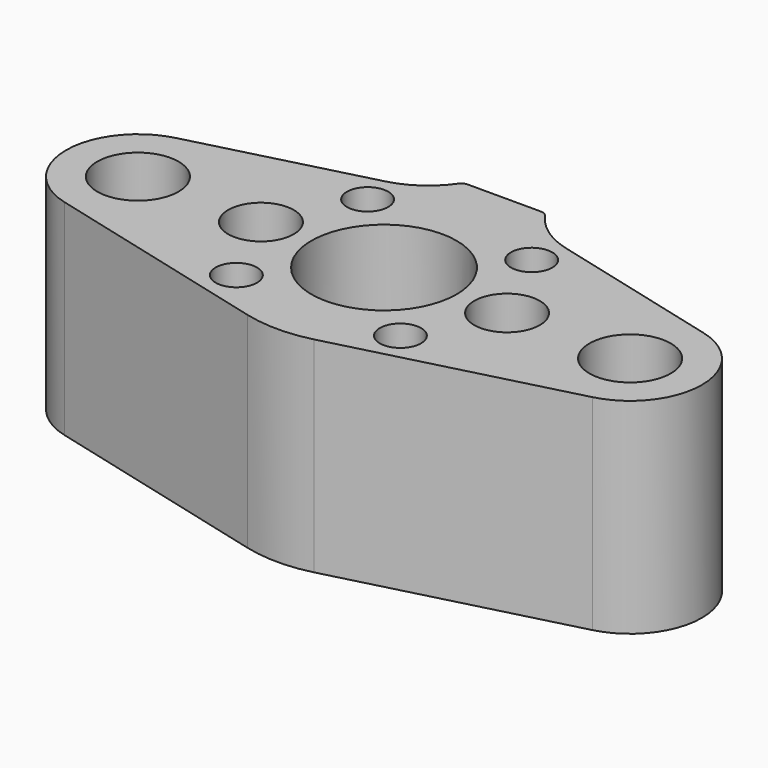
from build123d import *

# Parameters (mm, degrees)
F0_R        = 3.2004
F0_R_2      = 6.2992
F0_R_3      = 5.08
F0_R_4      = 11.2395
F1_DEPTH    = 31.75
F2_W        = 12.7
F2_H        = 5.1071889116
F3_DEPTH    = 31.75
F4_T1_DEPTH = 31.75
F5_R        = 1.27
F6_R        = 2.9845
F7_DEPTH    = 25.4


# Not quite as in the source:
# - a fillet or chamfer that OpenCascade refuses, or shapes differently, is made with other operations: its cross-section is extruded or revolved along the edge and cut away or added


with BuildPart() as f1:
    # F0 (on Top) → F1 (new body)
    with BuildSketch(Plane.XY):
        with BuildLine():
            Line((-5.159375, 19.9821734518), (-40.878125, 10.7596318587))
            ThreePointArc((-40.878125, 10.7596318587), (-49.2125, 0), (-40.878125, -10.7596318587))
            Line((-40.878125, -10.7596318587), (-5.159375, -19.9821734518))
            ThreePointArc((-5.159375, -19.9821734518), (0, -20.6375), (5.159375, -19.9821734518))
            Line((5.159375, -19.9821734518), (40.878125, -10.7596318587))
            ThreePointArc((40.878125, -10.7596318587), (49.2125, 0), (40.878125, 10.7596318587))
            Line((40.878125, 10.7596318587), (5.159375, 19.9821734518))
            ThreePointArc((5.159375, 19.9821734518), (0, 20.6375), (-5.159375, 19.9821734518))
        make_face()
        with Locations((-12.7, -12.7)):
            Circle(F0_R, mode=Mode.SUBTRACT)
        with Locations((12.7, -12.7)):
            Circle(F0_R, mode=Mode.SUBTRACT)
        with Locations((-38.1, 0)):
            Circle(F0_R_2, mode=Mode.SUBTRACT)
        with Locations((-19.05, 0)):
            Circle(F0_R_3, mode=Mode.SUBTRACT)
        with Locations((-12.7, 12.7)):
            Circle(F0_R, mode=Mode.SUBTRACT)
        Circle(F0_R_4, mode=Mode.SUBTRACT)
        with Locations((19.05, 0)):
            Circle(F0_R_3, mode=Mode.SUBTRACT)
        with Locations((38.1, 0)):
            Circle(F0_R_2, mode=Mode.SUBTRACT)
        with Locations((12.7, 12.7)):
            Circle(F0_R, mode=Mode.SUBTRACT)
    extrude(amount=F1_DEPTH)

    # F2 (on face) → F3 (join)
    with BuildSketch(Plane.XY.offset(31.75)):
        with Locations((0, 20.7509055442)):
            Rectangle(F2_W, F2_H)
    extrude(amount=-F3_DEPTH)

    # F4: fillet of radius 12.7 on 2 edges, made by hand

    # F4_s2 → F4_t1 (join)
    with BuildSketch(Plane.XY):
        with BuildLine():
            ThreePointArc((-13.9630832797, 17.7090657484), (-9.6168370541, 19.7724670423), (-6.35, 23.3045))
            Line((-6.35, 23.3045), (-6.35, 19.6747553987))
            Line((-6.35, 19.6747553987), (-13.9630832797, 17.7090657484))
        make_face()
        with BuildLine():
            ThreePointArc((13.9630832797, 17.7090657484), (9.6168370541, 19.7724670423), (6.35, 23.3045))
            Line((6.35, 23.3045), (6.35, 19.6747553987))
            Line((6.35, 19.6747553987), (13.9630832797, 17.7090657484))
        make_face()
    extrude(amount=F4_T1_DEPTH)

    # F5
    f5_edges = [f1.edges().sort_by_distance(p)[0] for p in [
        (-6.35, 23.3045, 15.875),
        (6.35, 23.3045, 15.875),
    ]]
    fillet(f5_edges, radius=F5_R)

    # F6 (on face) → F7 (cut)
    with BuildSketch(Plane(origin=(0, 23.3045, 0), x_dir=(-1, 0, 0), z_dir=(0, 1, 0))):
        with Locations((0, 15.875)):
            Circle(F6_R)
    extrude(amount=-F7_DEPTH, mode=Mode.SUBTRACT)


solid = f1.part
